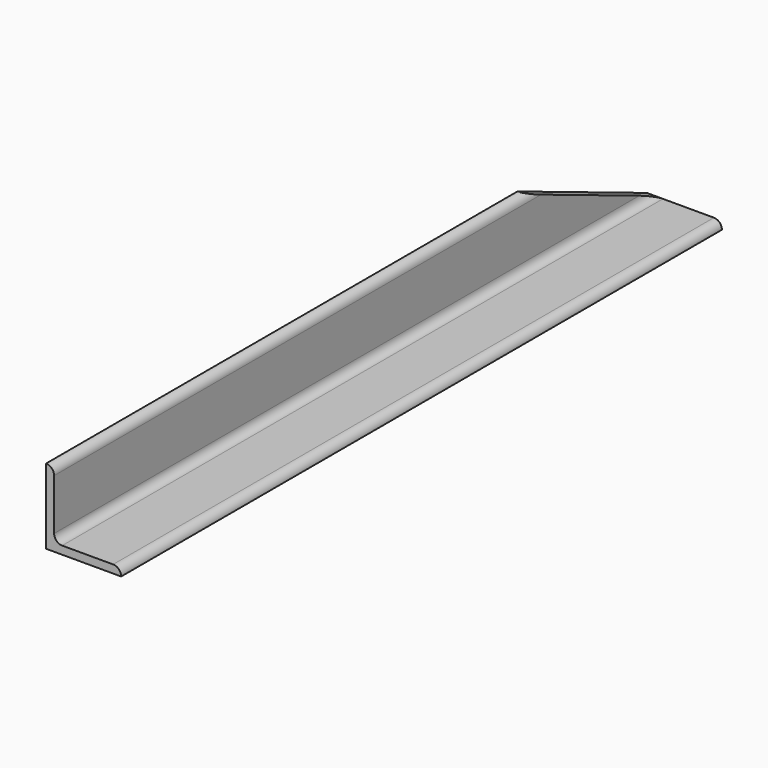
from build123d import *

# Parameters (mm, degrees)
F0_W     = 4.7625
F0_H     = 4.7625
F0_H_2   = 39.6875
F0_W_2   = 39.6875
F1_DEPTH = 222.25
F2_R     = 4.76249
F4_DEPTH = 25.4


# Not quite as in the source:
# - a fillet or chamfer is up to 0.001 mm smaller than in the source, because OpenCascade refuses the exact size


with BuildPart() as f1:
    # F0 (on Front) → F1 (new body, symmetric)
    with BuildSketch(Plane.XZ):
        with Locations((2.38125, 2.38125)):
            Rectangle(F0_W, F0_H)
        with Locations((2.38125, 24.60625)):
            Rectangle(F0_W, F0_H_2)
        with Locations((24.60625, 2.38125)):
            Rectangle(F0_W_2, F0_H)
    extrude(amount=F1_DEPTH, both=True)

    # F2 (radius 4.7625 in the source; OpenCascade refuses exactly that, so slightly less here)
    f2_edges = [f1.edges().sort_by_distance(p)[0] for p in [
        (4.7625, 0, 4.7625),
        (4.7625, 0, 44.45),
        (44.45, 0, 4.7625),
    ]]
    fillet(f2_edges, radius=F2_R)

    # F3 (on face) → F4 (cut)
    with BuildSketch(Plane(origin=(0, 0, 0), x_dir=(0, -1, 0), z_dir=(-1, 0, 0))):
        Polygon((-222.25, 44.45), (-222.25, 4.7625), (-126.4358992433, 44.45), align=None)
    extrude(amount=-F4_DEPTH, mode=Mode.SUBTRACT)


solid = f1.part
